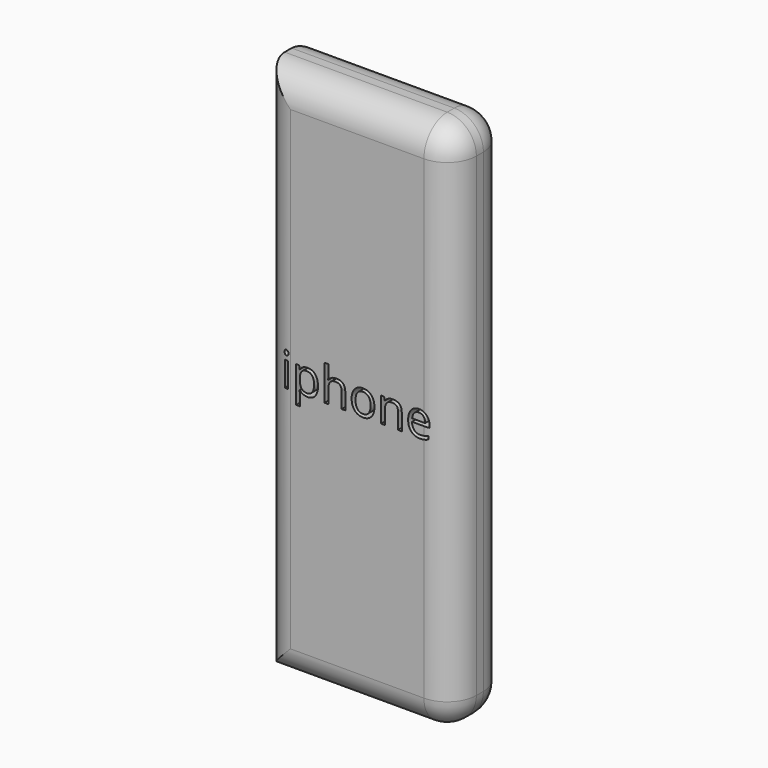
from build123d import *

# Parameters (mm, degrees)
F0_W         = 72.6124793291
F0_H         = 201.8705308437
F1_DEPTH     = 25.4
F2_R         = 11.0377844072
F3_TEXT_SIZE = 17.570062644
F4_DEPTH     = 37.338


# Not quite as in the source:
# - Text() gives the source's letters only with a copy of the font that has no kerning and outlines rounded to 1/6400 em; it was checked with that copy


with BuildPart() as f1:
    # F0 (on Front) → F1 (new body)
    with BuildSketch(Plane.XZ):
        with Locations((14.5993344486, -19.4134041667)):
            Rectangle(F0_W, F0_H)
    extrude(amount=F1_DEPTH)

    # F2
    f2_edges = [f1.edges().sort_by_distance(p)[0] for p in [
        (14.599334, -25.4, 81.521861),
        (14.599334, 0, 81.521861),
        (50.905574, -25.4, -19.413404),
        (50.905574, -12.7, -120.34867),
        (50.905574, -12.7, 81.521861),
        (50.905574, 0, -19.413404),
        (-21.706905, -25.4, -19.413404),
        (-21.706905, 0, -19.413404),
        (14.599334, 0, -120.34867),
        (14.599334, -25.4, -120.34867),
    ]]
    fillet(f2_edges, radius=F2_R)

    # F3 (on face) → F4 (cut)
    with BuildSketch(Plane.XZ.offset(25.4)):
        with Locations((-14.4846495241, -23.0991598219)):
            Text('iphone', F3_TEXT_SIZE, font='Open Sans', text_align=(TextAlign.LEFT, TextAlign.BOTTOM))
    extrude(amount=-F4_DEPTH, mode=Mode.SUBTRACT)


solid = f1.part
